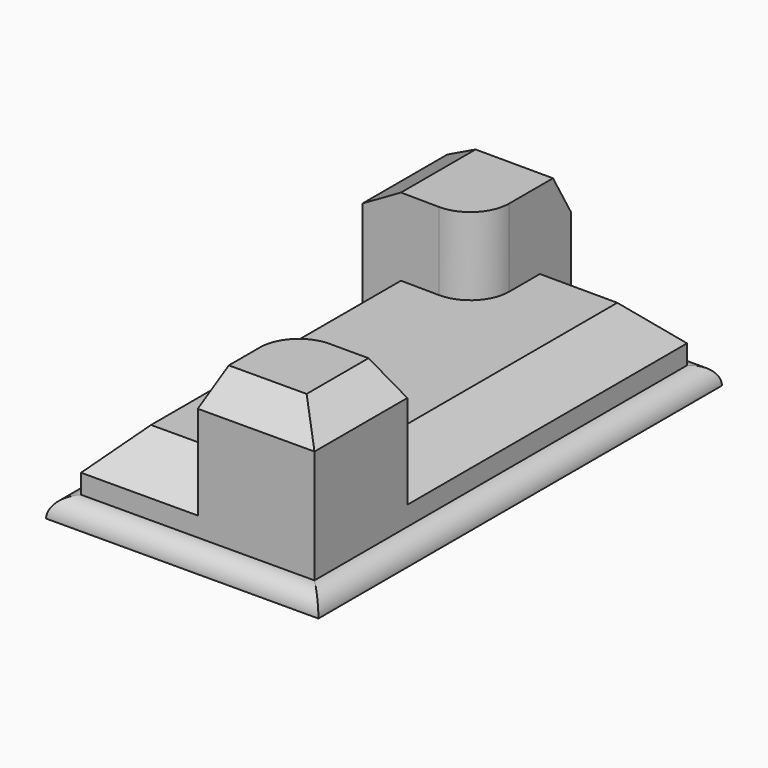
from build123d import *

# Parameters (mm, degrees)
F1_DEPTH    = 6.35
F2_DEPTH    = 25.4
F3_DEPTH    = 50.8
F4_R        = 6.34999
F5_SIZE     = 12.7
F6_C1_SIZE2 = 12.7
F6_C1_SIZE  = 7.3323484187
F6_C2_SIZE2 = 12.7
F6_C2_SIZE  = 7.3323484187
F6_C3_SIZE2 = 7.3323484187
F6_C3_SIZE  = 12.7
F6_C4_SIZE2 = 12.7
F6_C4_SIZE  = 7.3323484187


# Not quite as in the source:
# - a fillet or chamfer is up to 0.001 mm smaller than in the source, because OpenCascade refuses the exact size


with BuildPart() as f1:
    # F0 (on Top) → F1 (new body)
    with BuildSketch(Plane.XY):
        Polygon((-32.7964108223, 68.4432678408), (-121.6964108223, 68.7291226315), (-121.6964108223, -96.9018127685), (-32.7964108223, -96.6159616778), align=None)
        Polygon((-115.3464108223, 24.6241450903), (-115.3464108223, 62.3586716052), (-77.2464108223, 62.2361624092), (-39.1464108223, 62.1136532132), (-39.1464108223, -52.3088543971), (-39.1464108223, -90.2863467868), (-77.2464108223, -90.4088543971), (-115.3464108223, -90.5313620074), align=None, mode=Mode.SUBTRACT)
    extrude(amount=F1_DEPTH)

    # F0 (on Top) → F2 (join)
    with BuildSketch(Plane.XY):
        with BuildLine():
            Line((-90.1101133053, 24.2988232152), (-115.3464108223, 24.6241450903))
            Line((-115.3464108223, 24.6241450903), (-115.3464108223, -90.5313620074))
            Line((-115.3464108223, -90.5313620074), (-77.2464108223, -90.4088543971))
            Line((-77.2464108223, -90.4088543971), (-77.2464108223, -65.0088543971))
            ThreePointArc((-77.2464108223, -65.0088543971), (-73.5266669434, -56.028598276), (-64.5464108223, -52.3088543971))
            Line((-64.5464108223, -52.3088543971), (-39.1464108223, -52.3088543971))
            Line((-39.1464108223, -52.3088543971), (-39.1464108223, 62.1136532132))
            Line((-39.1464108223, 62.1136532132), (-77.2464108223, 62.2361624092))
            Line((-77.2464108223, 62.2361624092), (-77.2464108223, 36.9977681122))
            ThreePointArc((-77.2464108223, 36.9977681122), (-81.0242199909, 27.9598197407), (-90.1101133053, 24.2988232152))
        make_face()
    extrude(amount=F2_DEPTH)

    # F0 (on Top) → F3 (join)
    with BuildSketch(Plane.XY):
        with BuildLine():
            Line((-77.2464108223, -65.0088543971), (-77.2464108223, -90.4088543971))
            Line((-77.2464108223, -90.4088543971), (-39.1464108223, -90.2863467868))
            Line((-39.1464108223, -90.2863467868), (-39.1464108223, -52.3088543971))
            Line((-39.1464108223, -52.3088543971), (-64.5464108223, -52.3088543971))
            ThreePointArc((-64.5464108223, -52.3088543971), (-73.5266669434, -56.028598276), (-77.2464108223, -65.0088543971))
        make_face()
        with BuildLine():
            Line((-77.2464108223, 62.2361624092), (-115.3464108223, 62.3586716052))
            Line((-115.3464108223, 62.3586716052), (-115.3464108223, 24.6241450903))
            Line((-115.3464108223, 24.6241450903), (-90.1101133053, 24.2988232152))
            ThreePointArc((-90.1101133053, 24.2988232152), (-81.0242199909, 27.9598197407), (-77.2464108223, 36.9977681122))
            Line((-77.2464108223, 36.9977681122), (-77.2464108223, 62.2361624092))
        make_face()
    extrude(amount=F3_DEPTH)

    # F4 (radius 6.35 in the source; OpenCascade refuses exactly that, so slightly less here)
    f4_edges = [f1.edges().sort_by_distance(p)[0] for p in [
        (-77.246411, -96.758887, 6.35),
        (-32.796411, -14.086347, 6.35),
        (-77.246411, 68.586195, 6.35),
        (-121.696411, -14.086345, 6.35),
    ]]
    fillet(f4_edges, radius=F4_R)

    # F5
    f5_edges = [f1.edges().sort_by_distance(p)[0] for p in [
        (-96.296411, -90.470108, 25.4),
        (-39.146411, 4.902399, 25.4),
        (-115.346411, -32.953608, 25.4),
        (-58.196411, 62.174908, 25.4),
    ]]
    chamfer(f5_edges, length=F5_SIZE)

    # F6: chamfer of 12.7 x 7.3323484187 on 4 edges, made by hand

    # F6_c1
    f6_c1_edges = [f1.edges().sort_by_distance(p)[0] for p in [
        (-115.3464108223, 43.4914083477, 50.8),
    ]]
    f6_c1_side = f1.faces().sort_by_distance((-115.3464108223, 43.4914083477, 50.6533530316))[0]
    chamfer(f6_c1_edges, length=F6_C1_SIZE, length2=F6_C1_SIZE2, reference=f6_c1_side)

    # F6_c2
    f6_c2_edges = [f1.edges().sort_by_distance(p)[0] for p in [
        (-58.1964108223, -90.3476005919, 50.8),
    ]]
    f6_c2_side = f1.faces().sort_by_distance((-58.1964108223, -90.3476005919, 50.6533530316))[0]
    chamfer(f6_c2_edges, length=F6_C2_SIZE, length2=F6_C2_SIZE2, reference=f6_c2_side)

    # F6_c3
    f6_c3_edges = [f1.edges().sort_by_distance(p)[0] for p in [
        (-89.9464108223, 62.2769988079, 50.8),
    ]]
    f6_c3_side = f1.faces().sort_by_distance((-89.9464108223, 62.2769988079, 50.6533530316))[0]
    chamfer(f6_c3_edges, length=F6_C3_SIZE, length2=F6_C3_SIZE2, reference=f6_c3_side)

    # F6_c4
    f6_c4_edges = [f1.edges().sort_by_distance(p)[0] for p in [
        (-39.1464108223, -64.9475677659, 50.8),
    ]]
    f6_c4_side = f1.faces().sort_by_distance((-39.1464108223, -64.9475677659, 50.6533530316))[0]
    chamfer(f6_c4_edges, length=F6_C4_SIZE, length2=F6_C4_SIZE2, reference=f6_c4_side)


solid = f1.part
